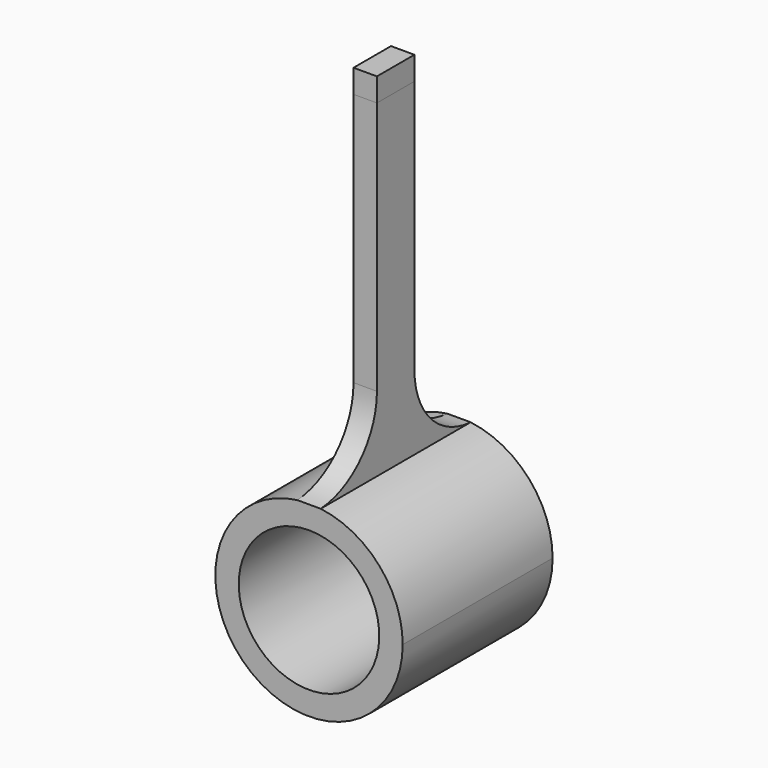
from build123d import *

# Parameters (mm, degrees)
F1_DEPTH    = 12.7
F3_DEPTH    = 25.4
F4_T1_DEPTH = 1.5875
F5_T1_DEPTH = 1.5875
F6_W        = 1.5875
F6_H        = 1.5875
F7_DEPTH    = 25.4
F8_W        = 1.5875
F8_H        = 3.175
F9_DEPTH    = 1.5875


# Not quite as in the source:
# - a fillet or chamfer that OpenCascade refuses, or shapes differently, is made with other operations: its cross-section is extruded or revolved along the edge and cut away or added


with BuildPart() as f1:
    # F0 (on Front) → F1 (new body)
    with BuildSketch(Plane.XZ):
        with BuildLine():
            Line((0.79375, 4.7625), (0, 4.7625))
            Line((0, 4.7625), (-0.79375, 4.7625))
            Line((-0.79375, 4.7625), (-0.79375, 6.3001953095))
            ThreePointArc((-0.79375, 6.3001953095), (-4.2001302063, -4.7625), (6.35, 0))
            ThreePointArc((6.35, 0), (4.7625, 4.2001302063), (0.79375, 6.3001953095))
            Line((0.79375, 6.3001953095), (0.79375, 4.7625))
        make_face()
        with BuildLine():
            ThreePointArc((0, 4.7625), (3.3675960454, 3.3675960454), (4.7625, 0))
            ThreePointArc((4.7625, 0), (-3.3675960454, -3.3675960454), (0, 4.7625))
        make_face(mode=Mode.SUBTRACT)
        with BuildLine():
            Line((-0.79375, 4.7625), (0, 4.7625))
            Line((0, 4.7625), (0.79375, 4.7625))
            Line((0.79375, 4.7625), (0.79375, 6.3001953095))
            ThreePointArc((0.79375, 6.3001953095), (0, 6.35), (-0.79375, 6.3001953095))
            Line((-0.79375, 6.3001953095), (-0.79375, 4.7625))
        make_face()
        with BuildLine():
            Line((-0.79375, 30.1625), (-0.79375, 6.3001953095))
            ThreePointArc((-0.79375, 6.3001953095), (0, 6.35), (0.79375, 6.3001953095))
            Line((0.79375, 6.3001953095), (0.79375, 30.1625))
            Line((0.79375, 30.1625), (-0.79375, 30.1625))
        make_face()
    extrude(amount=F1_DEPTH)

    # F2 (on face) → F3 (cut)
    with BuildSketch(Plane.YZ.offset(0.79375)):
        Polygon((-7.9375, 6.3001953095), (-7.9375, 30.1625), (-4.7625, 30.1625), (-4.7625, 6.3001953095), (8.4503721446, 6.3001953095), (8.4503721446, 42.4300841987), (-23.5275886953, 42.4300841987), (-23.5275886953, 6.3001953095), align=None)
    extrude(amount=-F3_DEPTH, mode=Mode.SUBTRACT)

    # F4: fillet of radius 5.08 on 1 edges, made by hand

    # F4_s2 → F4_t1 (join)
    with BuildSketch(Plane.YZ.offset(-0.79375)):
        with BuildLine():
            ThreePointArc((0, 6.3001953095), (-3.3851544532, 7.892225486), (-4.7625, 11.3702637262))
            Line((-4.7625, 11.3702637262), (-4.7625, 6.3001953095))
            Line((-4.7625, 6.3001953095), (0, 6.3001953095))
        make_face()
    extrude(amount=F4_T1_DEPTH)

    # F5: fillet of radius 5.08 on 1 edges, made by hand

    # F5_s2 → F5_t1 (join)
    with BuildSketch(Plane.YZ.offset(-0.79375)):
        with BuildLine():
            ThreePointArc((-7.9375, 11.3702637262), (-9.3148455468, 7.892225486), (-12.7, 6.3001953095))
            Line((-12.7, 6.3001953095), (-7.9375, 6.3001953095))
            Line((-7.9375, 6.3001953095), (-7.9375, 11.3702637262))
        make_face()
    extrude(amount=F5_T1_DEPTH)

    # F6 (on face) → F7 (cut)
    with BuildSketch(Plane(origin=(0, -4.7625, 0), x_dir=(-1, 0, 0), z_dir=(0, 1, 0))):
        with Locations((0, 29.36875)):
            Rectangle(F6_W, F6_H)
    extrude(amount=-F7_DEPTH, mode=Mode.SUBTRACT)


with BuildPart() as f9:
    # F8 (on face) → F9 (new body)
    with BuildSketch(Plane.XY.offset(28.575)):
        with Locations((0, -6.35)):
            Rectangle(F8_W, F8_H)
    extrude(amount=F9_DEPTH)


solid = Compound([f1.part, f9.part])
